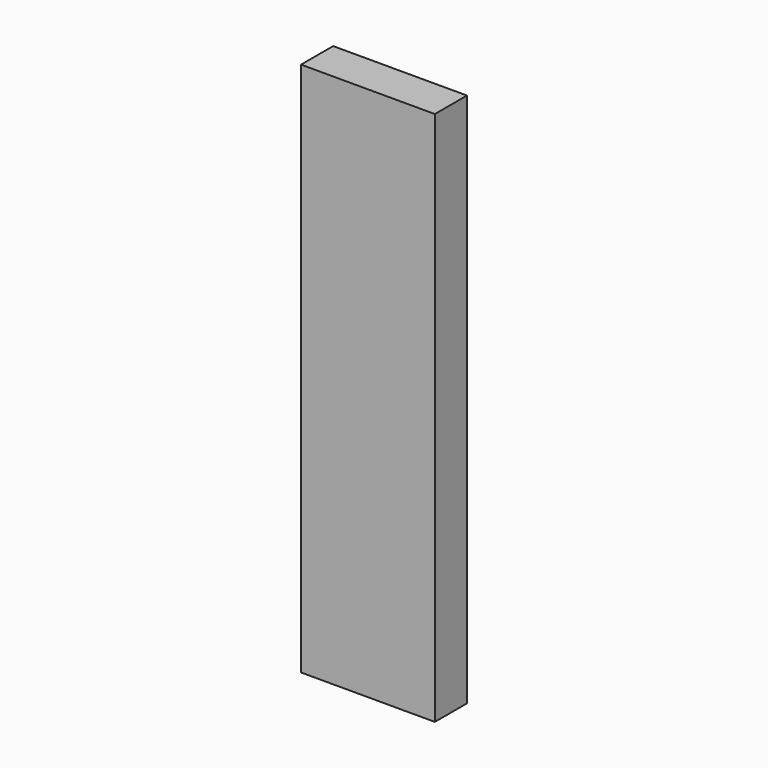
from build123d import *

# Parameters (mm, degrees)
F0_W     = 63.5
F0_H     = 254
F1_DEPTH = 19.05


# Not quite as in the source:
# - a length typed as a fraction of an inch, garbled in the dataset ("3 / 203.2 mm" for 3/8 in), is restored


with BuildPart() as f1:
    # F0 (on Front) → F1 (new body)
    with BuildSketch(Plane.XZ):
        Rectangle(F0_W, F0_H)
    extrude(amount=F1_DEPTH)


solid = f1.part
